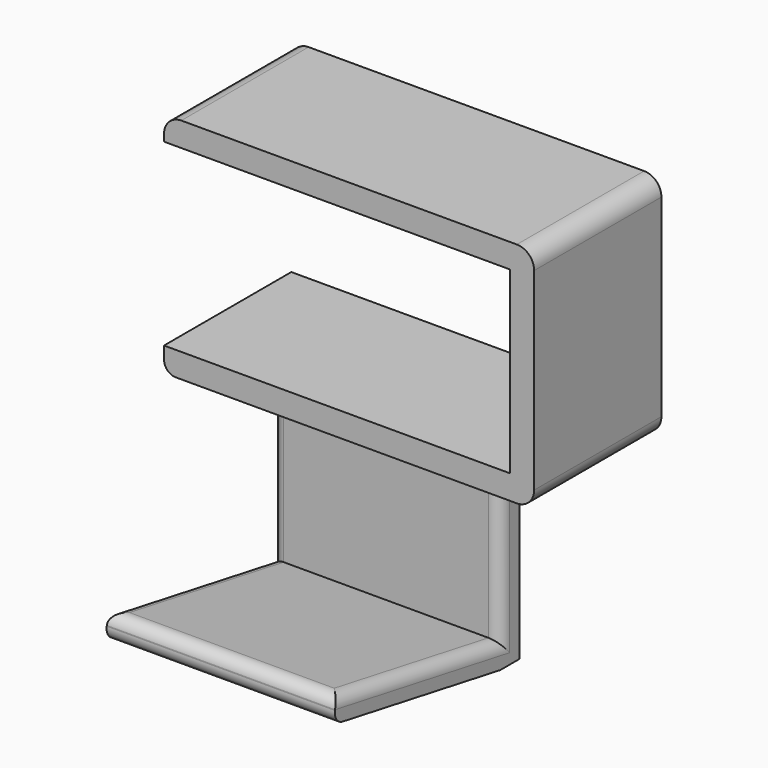
from build123d import *

# Parameters (mm, degrees)
F1_DEPTH = 23
F2_W     = 33
F2_H     = 3.5
F3_DEPTH = 35
F5_DEPTH = 33
F6_R     = 2.5
F7_R     = 1.7


with BuildPart() as f1:
    # F0 (on Front) → F1 (new body)
    with BuildSketch(Plane.XZ):
        Polygon((-53.5, 32.94), (-53.5, 29.44), (-3.5, 29.44), (-3.5, 3.5), (-53.5, 3.5), (-53.5, 0), (0, 0), (0, 32.94), align=None)
    extrude(amount=F1_DEPTH)

    # F2 (on face) → F3 (join)
    with BuildSketch(Plane(origin=(0, 0, 0), x_dir=(1, 0, 0), z_dir=(0, 0, -1))):
        with Locations((-37, 1.75)):
            Rectangle(F2_W, F2_H)
    extrude(amount=F3_DEPTH)

    # F4 (on face) → F5 (join, through all)
    with BuildSketch(Plane.YZ.offset(-20.5)):
        Polygon((-33.6520012122, -29.6833886639), (-3.5, -35), (-3.5, -31.4460068584), (-33.0442325904, -26.2365615284), align=None)
    extrude(amount=-F5_DEPTH)

    # F6
    f6_edges = [f1.edges().sort_by_distance(p)[0] for p in [
        (-53.5, -11.5, 32.94),
        (0, -11.5, 32.94),
        (0, -11.5, 0),
    ]]
    fillet(f6_edges, radius=F6_R)

    # F7
    f7_edges = [f1.edges().sort_by_distance(p)[0] for p in [
        (-37, -33.652001, -29.683389),
        (-37, -33.044233, -26.236562),
        (-20.5, -18.272116, -28.841284),
        (-53.5, -18.272116, -28.841284),
        (-20.5, -3.5, -15.723003),
        (-37, -3.5, 0),
        (-53.5, -13.25, 0),
        (-53.5, -3.5, -15.723003),
        (-20.5, -1.75, 0),
    ]]
    fillet(f7_edges, radius=F7_R)


solid = f1.part
